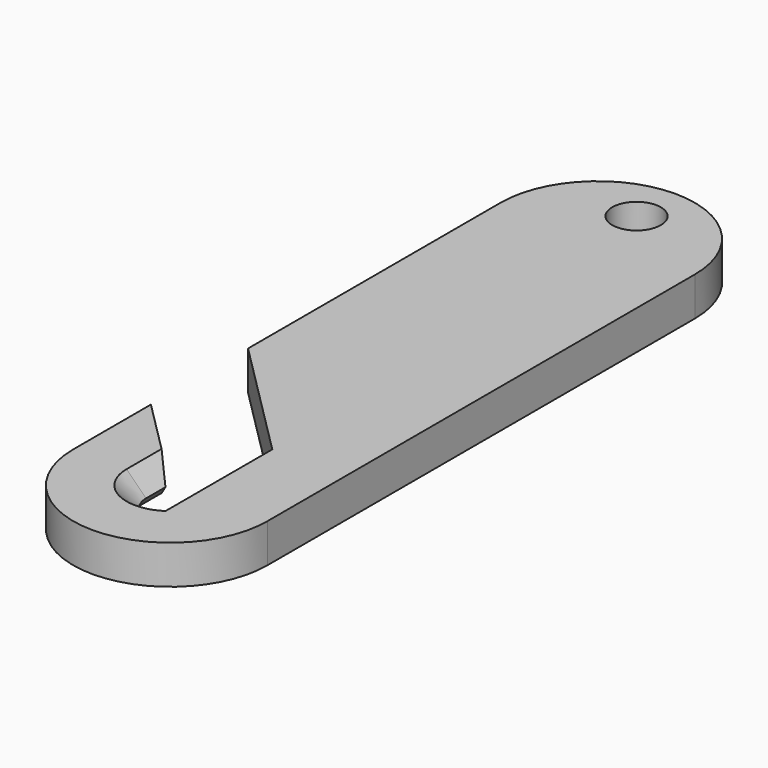
from build123d import *

# Parameters (mm, degrees)
F0_R     = 2.5
F1_DEPTH = 4
F2_SIZE  = 1.99999
F3_W     = 3.2302876376
F3_H     = 15.0867640845
F4_DEPTH = 4


# Not quite as in the source:
# - a fillet or chamfer is up to 0.001 mm smaller than in the source, because OpenCascade refuses the exact size


with BuildPart() as f1:
    # F0 (on Top) → F1 (new body)
    with BuildSketch(Plane.XY):
        with BuildLine():
            ThreePointArc((-6.116279643, 38.6264544598), (-16.116279643, 28.6264544598), (-26.116279643, 38.6264544598))
            Line((-26.116279643, 38.6264544598), (-26.116279643, 6.1264544598))
            Line((-26.116279643, 6.1264544598), (-16.116279643, -3.8735455402))
            Line((-16.116279643, -3.8735455402), (-13.616279643, -6.3735455402))
            Line((-13.616279643, -6.3735455402), (-13.616279643, -12.0434185212))
            Line((-13.616279643, -12.0434185212), (-13.616279643, -16.3735455402))
            Line((-13.616279643, -16.3735455402), (-13.616279643, -20.7036725591))
            ThreePointArc((-13.616279643, -20.7036725591), (-18.616279643, -20.7036725591), (-21.116279643, -16.3735455402))
            Line((-21.116279643, -16.3735455402), (-21.116279643, -11.3735455402))
            Line((-21.116279643, -11.3735455402), (-26.116279643, -6.3735455402))
            Line((-26.116279643, -6.3735455402), (-26.116279643, -16.3735455402))
            ThreePointArc((-26.116279643, -16.3735455402), (-16.116279643, -26.3735455402), (-6.116279643, -16.3735455402))
            Line((-6.116279643, -16.3735455402), (-6.116279643, 38.6264544598))
        make_face()
        with BuildLine():
            ThreePointArc((-6.116279643, 38.6264544598), (-16.116279643, 48.6264544598), (-26.116279643, 38.6264544598))
            ThreePointArc((-26.116279643, 38.6264544598), (-16.116279643, 28.6264544598), (-6.116279643, 38.6264544598))
        make_face()
        with Locations((-16.116279643, 43.6264544598)):
            Circle(F0_R, mode=Mode.SUBTRACT)
        with BuildLine():
            Line((-13.616279643, -20.7036725591), (-13.616279643, -16.3735455402))
            ThreePointArc((-13.616279643, -16.3735455402), (-16.116279643, -18.8735455402), (-18.616279643, -16.3735455402))
            Line((-18.616279643, -16.3735455402), (-18.616279643, -13.8735455402))
            Line((-18.616279643, -13.8735455402), (-21.116279643, -11.3735455402))
            Line((-21.116279643, -11.3735455402), (-21.116279643, -16.3735455402))
            ThreePointArc((-21.116279643, -16.3735455402), (-18.616279643, -20.7036725591), (-13.616279643, -20.7036725591))
        make_face()
    extrude(amount=F1_DEPTH)

    # F2 (size 2 in the source; OpenCascade refuses exactly that, so slightly less here)
    f2_edges = [f1.edges().sort_by_distance(p)[0] for p in [
        (-16.11628, -18.873546, 4),
        (-18.61628, -15.123546, 4),
        (-16.11628, -18.873546, 0),
    ]]
    chamfer(f2_edges, length=F2_SIZE)

    # F3 (on face) → F4 (join)
    with BuildSketch(Plane.XY.offset(4)):
        with Locations((-12.0011358242, -13.9169275824)):
            Rectangle(F3_W, F3_H)
    extrude(amount=-F4_DEPTH)


solid = f1.part
